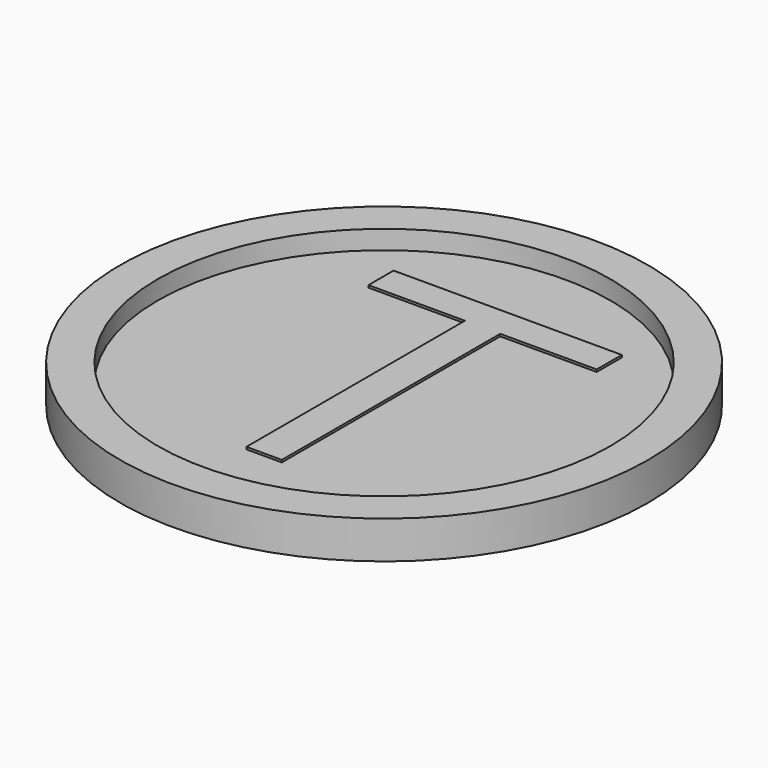
from build123d import *

# Parameters (mm, degrees)
F0_R         = 44.45
F1_DEPTH     = 6.35
F3_R         = 38.1
F4_DEPTH     = 3.175
F3_TEXT_SIZE = 71.8298812483
F5_DEPTH     = 2.794


# Not quite as in the source:
# - a feature names something its author has since deleted; it is built from what else it names
# - Text() gives the source's letters only with a copy of the font that has no kerning and outlines rounded to 1/6400 em; it was checked with that copy


with BuildPart() as f1:
    # F0 (on Top) → F1 (new body)
    with BuildSketch(Plane.XY):
        Circle(F0_R)
    extrude(amount=F1_DEPTH)

    # F3 (on offset) → F4 (cut)
    with BuildSketch(Plane.XY.offset(6.35)):
        Circle(F3_R)
        Polygon((3.4609341342, 20.1235901685), (3.4609341342, -25.8587572494), (-2.4987013256, -25.8587572494), (-2.4987013256, 20.1235901685), (-18.7389885391, 20.1235901685), (-18.7389885391, 25.4210439105), (19.7012213477, 25.4210439105), (19.7012213477, 20.1235901685), align=None, mode=Mode.SUBTRACT)
    extrude(amount=-F4_DEPTH, mode=Mode.SUBTRACT)

    # F3 (on offset) → F5 (cut)
    with BuildSketch(Plane.XY.offset(6.35)):
        with Locations((-19.3675, -25.8587572494)):
            Text('T', F3_TEXT_SIZE, font='Open Sans', text_align=(TextAlign.LEFT, TextAlign.BOTTOM))
    extrude(amount=-F5_DEPTH, mode=Mode.SUBTRACT)


solid = f1.part
